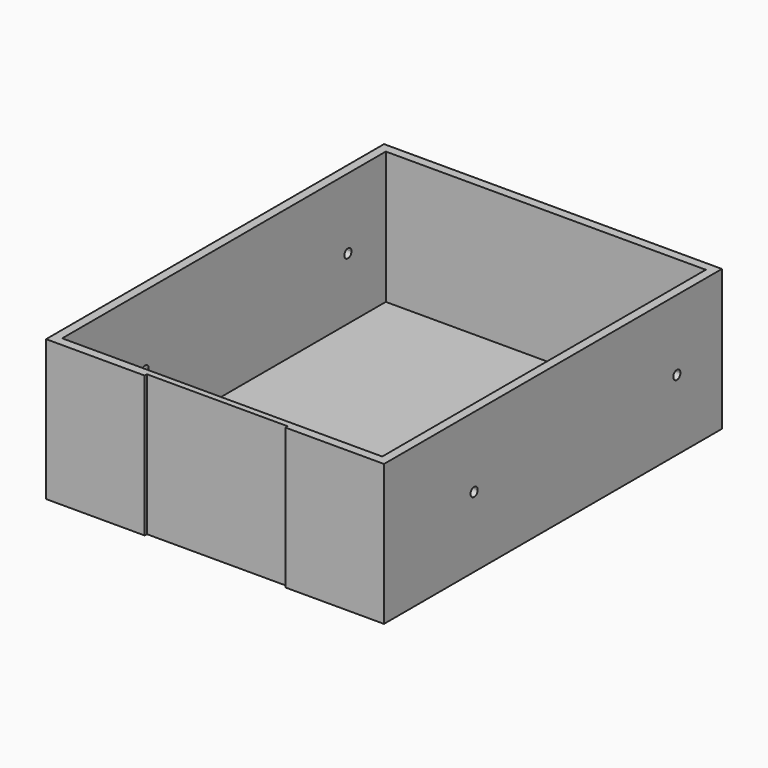
from build123d import *

# Parameters (mm, degrees)
F0_W     = 113.645
F0_H     = 3.18
F0_W_2   = 3.175
F0_H_2   = 143.64
F0_W_3   = 3.18
F1_DEPTH = 50
F2_W     = 113.64
F2_H     = 143.64
F3_DEPTH = 47
F5_DEPTH = 120.001
F6_W     = 50
F6_H     = 50
F7_DEPTH = 1


with BuildPart() as f1:
    # F0 (on Top) → F1 (new body)
    with BuildSketch(Plane.XY):
        with Locations((-10.0610243238, 113.2212999272)):
            Rectangle(F0_W, F0_H)
        with Locations((-68.4710243238, 113.2212999272)):
            Rectangle(F0_W_2, F0_H)
        with Locations((-68.4710243238, 39.8112999272)):
            Rectangle(F0_W_2, F0_H_2)
        with Locations((-10.0610243238, -33.5987000728)):
            Rectangle(F0_W, F0_H)
        with Locations((48.3514756762, 39.8112999272)):
            Rectangle(F0_W_3, F0_H_2)
        with Locations((48.3514756762, -33.5987000728)):
            Rectangle(F0_W_3, F0_H)
        with Locations((48.3514756762, 113.2212999272)):
            Rectangle(F0_W_3, F0_H)
        with Locations((-68.4710243238, -33.5987000728)):
            Rectangle(F0_W_2, F0_H)
        with Locations((-10.0610243238, 39.8112999272)):
            Rectangle(F0_W, F0_H_2)
    extrude(amount=F1_DEPTH)

    # F2 (on face) → F3 (cut)
    with BuildSketch(Plane.XY.offset(50)):
        with Locations((-10.0585243238, 39.8112999272)):
            Rectangle(F2_W, F2_H)
    extrude(amount=-F3_DEPTH, mode=Mode.SUBTRACT)

    # F4 (on face) → F5 (cut, through all)
    with BuildSketch(Plane.YZ.offset(49.9414756762)):
        with BuildLine():
            ThreePointArc((6.4012999272, 25), (5.9355997093, 26.1242997821), (4.8112999272, 26.59))
            Line((4.8112999272, 26.59), (4.8112999272, 23.41))
            ThreePointArc((4.8112999272, 23.41), (5.9355997093, 23.8757002179), (6.4012999272, 25))
        make_face()
        with BuildLine():
            Line((4.8112999272, 23.41), (4.8112999272, 26.59))
            ThreePointArc((4.8112999272, 26.59), (3.2212999272, 25), (4.8112999272, 23.41))
        make_face()
        with BuildLine():
            ThreePointArc((96.4012999272, 25), (95.9355997093, 26.1242997821), (94.8112999272, 26.59))
            Line((94.8112999272, 26.59), (94.8112999272, 23.41))
            ThreePointArc((94.8112999272, 23.41), (95.9355997093, 23.8757002179), (96.4012999272, 25))
        make_face()
        with BuildLine():
            Line((94.8112999272, 23.41), (94.8112999272, 26.59))
            ThreePointArc((94.8112999272, 26.59), (93.2212999272, 25), (94.8112999272, 23.41))
        make_face()
    extrude(amount=-F5_DEPTH, mode=Mode.SUBTRACT)

    # F6 (on face) → F7 (cut)
    with BuildSketch(Plane.XZ.offset(35.1887000728)):
        with Locations((-10.0585243238, 25)):
            Rectangle(F6_W, F6_H)
    extrude(amount=-F7_DEPTH, mode=Mode.SUBTRACT)


solid = f1.part
